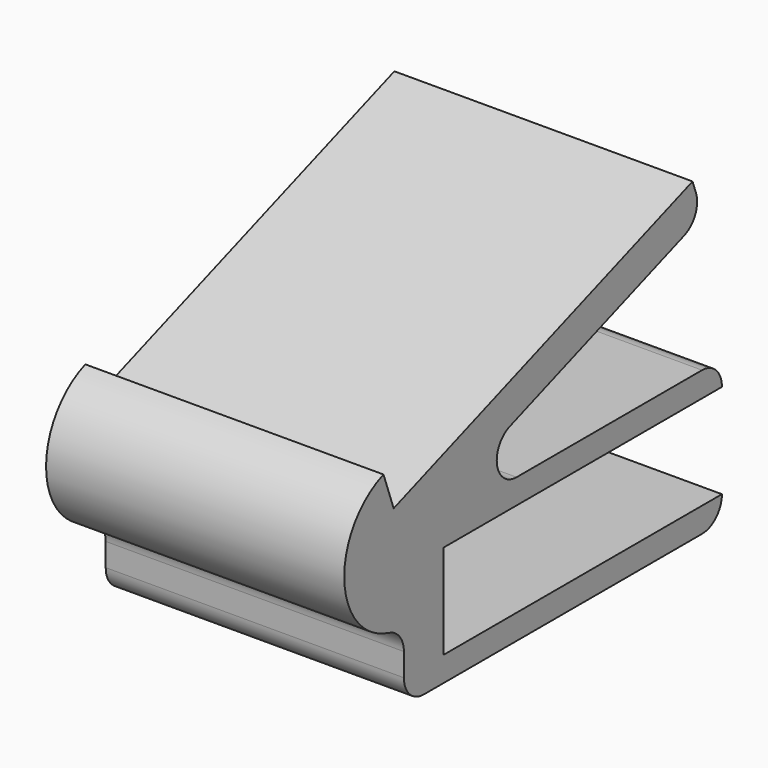
from build123d import *

# Parameters (mm, degrees)
F1_DEPTH = 60
F2_R     = 4.99999


# Not quite as in the source:
# - a fillet or chamfer is up to 0.001 mm smaller than in the source, because OpenCascade refuses the exact size


with BuildPart() as f1:
    # F0 (on Right) → F1 (new body)
    with BuildSketch(Plane.YZ):
        Polygon((-80, 0), (0, 0), (0, 5), (-70, 5), (-70, 24), (0, 24), (0, 29), (-80, 29), (-80, 14), align=None)
        with BuildLine():
            ThreePointArc((-85.1303021499, 43.0953893118), (-94.7721162952, 26.395277335), (-80, 14))
            Line((-80, 14), (-80, 29))
            Line((-80, 29), (-82.5651510749, 36.0476946559))
            Line((-82.5651510749, 36.0476946559), (-85.1303021499, 43.0953893118))
        make_face()
        Polygon((-82.5651510749, 36.0476946559), (-80, 29), (-4.8245903371, 56.3616114661), (-7.3897414121, 63.4093061219), align=None)
    extrude(amount=F1_DEPTH)

    # F2 (radius 5 in the source; OpenCascade refuses exactly that, so slightly less here)
    f2_edges = [f1.edges().sort_by_distance(p)[0] for p in [
        (30, -80, 29),
        (30, -80, 14),
        (30, -80, 0),
        (30, 0, 0),
        (30, 0, 29),
        (30, -4.82459, 56.361611),
    ]]
    fillet(f2_edges, radius=F2_R)


solid = f1.part
